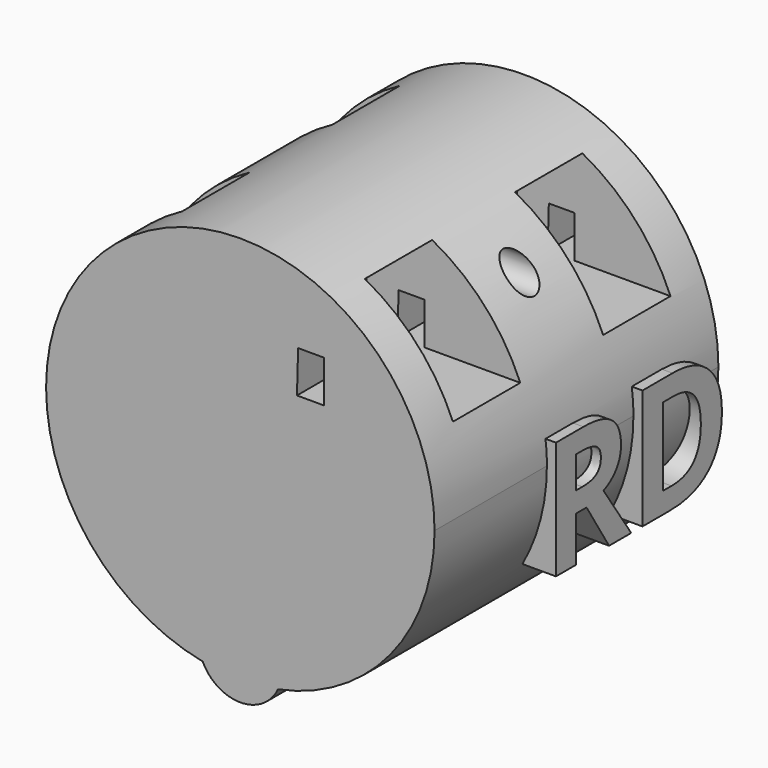
from build123d import *

# Parameters (mm, degrees)
F0_R          = 76.2
F1_DEPTH      = 69.596
F3_W          = 33.02
F3_H          = 38.1
F4_DEPTH      = 170.434
F5_W          = 20.2989353982
F5_H          = 62.2236525431
F6_DEPTH      = 135.128
F7_R          = 16.3523895673
F8_DEPTH      = 69.596
F10_DEPTH     = 136.652
F11_TEXT_SIZE = 65.7688179571
F12_DEPTH     = 25.908
F13_TEXT_SIZE = 64.6965009057
F14_DEPTH     = 13.97
F15_R         = 6.1452455288
F16_DEPTH     = 82.804


# Not quite as in the source:
# - Text() gives the source's letters only with a copy of the font that has no kerning and outlines rounded to 1/6400 em; it was checked with that copy


with BuildPart() as f1:
    # F0 (on Front) → F1 (new body, symmetric)
    with BuildSketch(Plane.XZ):
        Circle(F0_R)
    extrude(amount=F1_DEPTH, both=True)

    # F3 (on offset) → F4 (cut)
    with BuildSketch(Plane.YZ.offset(79.756)):
        with Locations((-36.83, 48.1987432095)):
            Rectangle(F3_W, F3_H)
        with Locations((36.83, 48.1987432095)):
            Rectangle(F3_W, F3_H)
    extrude(amount=-F4_DEPTH, mode=Mode.SUBTRACT)

    # F5 (on face) → F6 (join)
    with BuildSketch(Plane(origin=(0, 69.596, 0), x_dir=(-1, 0, 0), z_dir=(0, 1, 0))):
        with Locations((0, 44.4092191756)):
            Rectangle(F5_W, F5_H)
    extrude(amount=-F6_DEPTH)

    # F7 (on Front) → F8 (join, symmetric)
    with BuildSketch(Plane.XZ):
        with Locations((0, -67.7437782288)):
            Circle(F7_R)
    extrude(amount=F8_DEPTH, both=True)

    # F9 (on face) → F10 (cut, symmetric)
    with BuildSketch(Plane(origin=(0, -53.34, 0), x_dir=(-1, 0, 0), z_dir=(0, 1, 0))):
        Polygon((-32.8352851158, 45.6587432095), (-32.8352851158, 29.1487432095), (-22.2161393613, 29.1487432095), (-22.6752851158, 45.6587432095), align=None)
    extrude(amount=F10_DEPTH, both=True, mode=Mode.SUBTRACT)

    # F11 (on offset) → F12 (join)
    with BuildSketch(Plane.YZ.offset(79.756)):
        with Locations((22.0039598644, -37.0183624327)):
            Text('D', F11_TEXT_SIZE, font='Open Sans', font_style=FontStyle.BOLD, text_align=(TextAlign.LEFT, TextAlign.BOTTOM))
    extrude(amount=-F12_DEPTH)

    # F13 (on offset) → F14 (join)
    with BuildSketch(Plane.YZ.offset(79.756)):
        with Locations((-20.3241454437, -37.0183624327)):
            Text('R', F13_TEXT_SIZE, font='Open Sans', font_style=FontStyle.BOLD, text_align=(TextAlign.LEFT, TextAlign.BOTTOM))
    extrude(amount=-F14_DEPTH)

    # F15 (on offset) → F16 (cut)
    with BuildSketch(Plane.YZ.offset(79.756)):
        with Locations((0, 53.5302422941)):
            Circle(F15_R)
    extrude(amount=-F16_DEPTH, mode=Mode.SUBTRACT)


solid = f1.part
